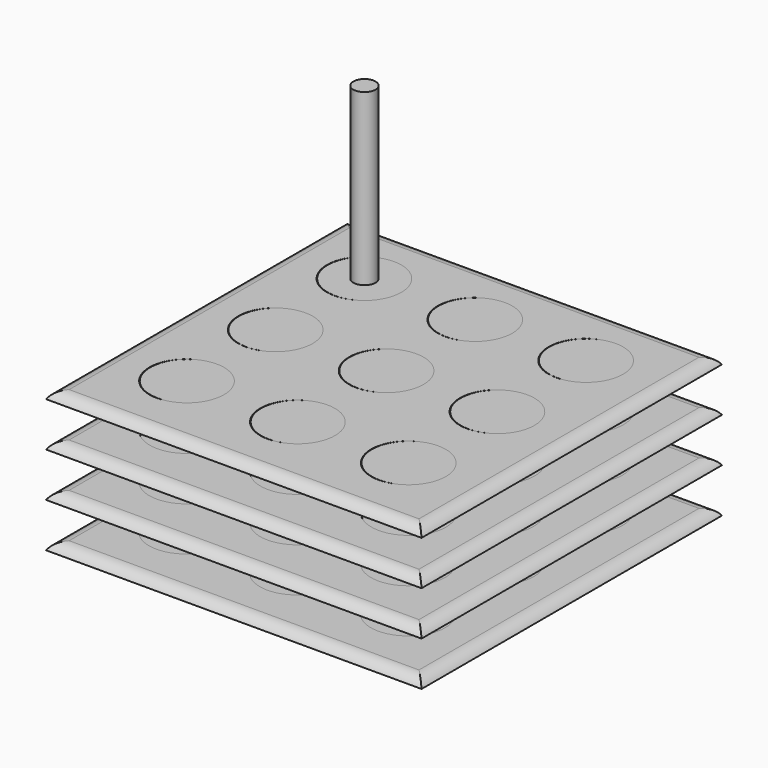
from build123d import *

# Parameters (mm, degrees)
F0_W        = 50.8
F0_H        = 50.8
F1_DEPTH    = 1
F2_T1_DEPTH = 59.4602540378
F2_T3_DEPTH = 59.4602540378
F4_D        = 10
F4_DEPTH    = 1
F4_TIP      = 3.0043030951
F6_R        = 5.0378850753
F7_DEPTH    = 1
F10_R       = 5.0007120409
F11_DEPTH   = 1
F14_R       = 5.0415091702
F15_DEPTH   = 1
F18_R       = 5.001829943
F19_DEPTH   = 1
F20_R       = 1.5
F21_DEPTH   = 40


# Not quite as in the source:
# - a fillet or chamfer that OpenCascade refuses, or shapes differently, is made with other operations: its cross-section is extruded or revolved along the edge and cut away or added


with BuildPart() as f1:
    # F0 (on Top) → F1 (new body)
    with BuildSketch(Plane.XY):
        with Locations((4.2530756999, 25.4)):
            Rectangle(F0_W, F0_H)
    extrude(amount=F1_DEPTH)

    # F2: fillet of radius 2 on 4 edges, made by hand

    # F2_s2 → F2_t1 (cut)
    with BuildSketch(Plane.YZ.offset(-25.477051319)):
        with BuildLine():
            ThreePointArc((0, 0), (0.7320508076, 0.7320508076), (1.7320508076, 1))
            Line((1.7320508076, 1), (0, 1))
            Line((0, 1), (0, 0))
        make_face()
        with BuildLine():
            ThreePointArc((50.8, 0), (50.0679491924, 0.7320508076), (49.0679491924, 1))
            Line((49.0679491924, 1), (50.8, 1))
            Line((50.8, 1), (50.8, 0))
        make_face()
    extrude(amount=F2_T1_DEPTH, mode=Mode.SUBTRACT)

    # F2_s4 → F2_t3 (cut)
    with BuildSketch(Plane.XZ.offset(-55.1301270189)):
        with BuildLine():
            ThreePointArc((29.6530756999, 0), (28.9210248923, 0.7320508076), (27.9210248923, 1))
            Line((27.9210248923, 1), (29.6530756999, 1))
            Line((29.6530756999, 1), (29.6530756999, 0))
        make_face()
        with BuildLine():
            ThreePointArc((-21.1469243001, 0), (-20.4148734925, 0.7320508076), (-19.4148734925, 1))
            Line((-19.4148734925, 1), (-21.1469243001, 1))
            Line((-21.1469243001, 1), (-21.1469243001, 0))
        make_face()
    extrude(amount=F2_T3_DEPTH, mode=Mode.SUBTRACT)

    # F4
    with Locations(Plane.XY.offset(1)):
        with Locations((19.036982879, 41.0148405656), (19.036982879, 26.0148405656), (19.036982879, 11.0148405656), (4.036982879, 11.0148405656), (4.036982879, 26.0148405656), (4.036982879, 41.0148405656), (-10.963017121, 41.0148405656), (-10.963017121, 26.0148405656), (-10.963017121, 11.0148405656)):
            Hole(F4_D / 2, depth=F4_DEPTH)
            with Locations((0, 0, -(F4_DEPTH + F4_TIP / 2))):  # 118° drill point
                Cone(0, F4_D / 2, F4_TIP, mode=Mode.SUBTRACT)


with BuildPart() as f7:
    # F6 (on offset) → F7 (new body)
    with BuildSketch(Plane.XY.offset(1)):
        with Locations((-10.9860114753, 41.0153977573)):
            Circle(F6_R)
    extrude(amount=-F7_DEPTH)


with BuildPart() as f7b:
    # F6 (on offset) → F7, piece 2 (new body)
    with BuildSketch(Plane.XY.offset(1)):
        with Locations((4.0139885247, 41.0153977573)):
            Circle(F6_R)
    extrude(amount=-F7_DEPTH)


with BuildPart() as f7c:
    # F6 (on offset) → F7, piece 3 (new body)
    with BuildSketch(Plane.XY.offset(1)):
        with Locations((19.0139885247, 41.0153977573)):
            Circle(F6_R)
    extrude(amount=-F7_DEPTH)


with BuildPart() as f7d:
    # F6 (on offset) → F7, piece 4 (new body)
    with BuildSketch(Plane.XY.offset(1)):
        with Locations((-10.9860114753, 26.0153977573)):
            Circle(F6_R)
    extrude(amount=-F7_DEPTH)


with BuildPart() as f7e:
    # F6 (on offset) → F7, piece 5 (new body)
    with BuildSketch(Plane.XY.offset(1)):
        with Locations((4.0139885247, 26.0153977573)):
            Circle(F6_R)
    extrude(amount=-F7_DEPTH)


with BuildPart() as f7f:
    # F6 (on offset) → F7, piece 6 (new body)
    with BuildSketch(Plane.XY.offset(1)):
        with Locations((19.0139885247, 26.0153977573)):
            Circle(F6_R)
    extrude(amount=-F7_DEPTH)


with BuildPart() as f7g:
    # F6 (on offset) → F7, piece 7 (new body)
    with BuildSketch(Plane.XY.offset(1)):
        with Locations((-10.9860114753, 11.0153977573)):
            Circle(F6_R)
    extrude(amount=-F7_DEPTH)


with BuildPart() as f7h:
    # F6 (on offset) → F7, piece 8 (new body)
    with BuildSketch(Plane.XY.offset(1)):
        with Locations((4.0139885247, 11.0153977573)):
            Circle(F6_R)
    extrude(amount=-F7_DEPTH)


with BuildPart() as f7i:
    # F6 (on offset) → F7, piece 9 (new body)
    with BuildSketch(Plane.XY.offset(1)):
        with Locations((19.0139885247, 11.0153977573)):
            Circle(F6_R)
    extrude(amount=-F7_DEPTH)


with BuildPart() as f8_1:
    # F8: copy of F1
    add(f1.part.moved(Location((0, 0, 6))))


with BuildPart() as f11:
    # F10 (on offset) → F11 (new body)
    with BuildSketch(Plane.XY.offset(7)):
        with Locations((19.0628959137, 40.9449415705)):
            Circle(F10_R)
    extrude(amount=-F11_DEPTH)


with BuildPart() as f11b:
    # F10 (on offset) → F11, piece 2 (new body)
    with BuildSketch(Plane.XY.offset(7)):
        with Locations((19.0628959137, 25.9449415705)):
            Circle(F10_R)
    extrude(amount=-F11_DEPTH)


with BuildPart() as f11c:
    # F10 (on offset) → F11, piece 3 (new body)
    with BuildSketch(Plane.XY.offset(7)):
        with Locations((19.0628959137, 10.9449415705)):
            Circle(F10_R)
    extrude(amount=-F11_DEPTH)


with BuildPart() as f11d:
    # F10 (on offset) → F11, piece 4 (new body)
    with BuildSketch(Plane.XY.offset(7)):
        with Locations((4.0628959137, 40.9449415705)):
            Circle(F10_R)
    extrude(amount=-F11_DEPTH)


with BuildPart() as f11e:
    # F10 (on offset) → F11, piece 5 (new body)
    with BuildSketch(Plane.XY.offset(7)):
        with Locations((4.0628959137, 25.9449415705)):
            Circle(F10_R)
    extrude(amount=-F11_DEPTH)


with BuildPart() as f11f:
    # F10 (on offset) → F11, piece 6 (new body)
    with BuildSketch(Plane.XY.offset(7)):
        with Locations((4.0628959137, 10.9449415705)):
            Circle(F10_R)
    extrude(amount=-F11_DEPTH)


with BuildPart() as f11g:
    # F10 (on offset) → F11, piece 7 (new body)
    with BuildSketch(Plane.XY.offset(7)):
        with Locations((-10.9371040863, 10.9449415705)):
            Circle(F10_R)
    extrude(amount=-F11_DEPTH)


with BuildPart() as f11h:
    # F10 (on offset) → F11, piece 8 (new body)
    with BuildSketch(Plane.XY.offset(7)):
        with Locations((-10.9371040863, 25.9449415705)):
            Circle(F10_R)
    extrude(amount=-F11_DEPTH)


with BuildPart() as f11i:
    # F10 (on offset) → F11, piece 9 (new body)
    with BuildSketch(Plane.XY.offset(7)):
        with Locations((-10.9371040863, 40.9449415705)):
            Circle(F10_R)
    extrude(amount=-F11_DEPTH)


with BuildPart() as f12_1:
    # F12: copy of F8_1
    add(f8_1.part.moved(Location((0, 0, 6))))


with BuildPart() as f15:
    # F14 (on offset) → F15 (new body)
    with BuildSketch(Plane.XY.offset(13)):
        with Locations((-10.9040877064, 41.0306417219)):
            Circle(F14_R)
    extrude(amount=-F15_DEPTH)


with BuildPart() as f15b:
    # F14 (on offset) → F15, piece 2 (new body)
    with BuildSketch(Plane.XY.offset(13)):
        with Locations((-10.9040877064, 26.0306417219)):
            Circle(F14_R)
    extrude(amount=-F15_DEPTH)


with BuildPart() as f15c:
    # F14 (on offset) → F15, piece 3 (new body)
    with BuildSketch(Plane.XY.offset(13)):
        with Locations((-10.9040877064, 11.0306417219)):
            Circle(F14_R)
    extrude(amount=-F15_DEPTH)


with BuildPart() as f15d:
    # F14 (on offset) → F15, piece 4 (new body)
    with BuildSketch(Plane.XY.offset(13)):
        with Locations((4.0959122936, 41.0306417219)):
            Circle(F14_R)
    extrude(amount=-F15_DEPTH)


with BuildPart() as f15e:
    # F14 (on offset) → F15, piece 5 (new body)
    with BuildSketch(Plane.XY.offset(13)):
        with Locations((4.0959122936, 26.0306417219)):
            Circle(F14_R)
    extrude(amount=-F15_DEPTH)


with BuildPart() as f15f:
    # F14 (on offset) → F15, piece 6 (new body)
    with BuildSketch(Plane.XY.offset(13)):
        with Locations((4.0959122936, 11.0306417219)):
            Circle(F14_R)
    extrude(amount=-F15_DEPTH)


with BuildPart() as f15g:
    # F14 (on offset) → F15, piece 7 (new body)
    with BuildSketch(Plane.XY.offset(13)):
        with Locations((19.0959122936, 41.0306417219)):
            Circle(F14_R)
    extrude(amount=-F15_DEPTH)


with BuildPart() as f15h:
    # F14 (on offset) → F15, piece 8 (new body)
    with BuildSketch(Plane.XY.offset(13)):
        with Locations((19.0959122936, 26.0306417219)):
            Circle(F14_R)
    extrude(amount=-F15_DEPTH)


with BuildPart() as f15i:
    # F14 (on offset) → F15, piece 9 (new body)
    with BuildSketch(Plane.XY.offset(13)):
        with Locations((19.0959122936, 11.0306417219)):
            Circle(F14_R)
    extrude(amount=-F15_DEPTH)


with BuildPart() as f16_1:
    # F16: copy of F12_1
    add(f12_1.part.moved(Location((0, 0, 6))))


with BuildPart() as f19:
    # F18 (on offset) → F19 (new body)
    with BuildSketch(Plane.XY.offset(19)):
        with Locations((-10.9060970124, 41.0428672295)):
            Circle(F18_R)
    extrude(amount=-F19_DEPTH)


with BuildPart() as f19b:
    # F18 (on offset) → F19, piece 2 (new body)
    with BuildSketch(Plane.XY.offset(19)):
        with Locations((-10.9060970124, 26.0428672295)):
            Circle(F18_R)
    extrude(amount=-F19_DEPTH)


with BuildPart() as f19c:
    # F18 (on offset) → F19, piece 3 (new body)
    with BuildSketch(Plane.XY.offset(19)):
        with Locations((-10.9060970124, 11.0428672295)):
            Circle(F18_R)
    extrude(amount=-F19_DEPTH)


with BuildPart() as f19d:
    # F18 (on offset) → F19, piece 4 (new body)
    with BuildSketch(Plane.XY.offset(19)):
        with Locations((4.0939029876, 41.0428672295)):
            Circle(F18_R)
    extrude(amount=-F19_DEPTH)


with BuildPart() as f19e:
    # F18 (on offset) → F19, piece 5 (new body)
    with BuildSketch(Plane.XY.offset(19)):
        with Locations((4.0939029876, 26.0428672295)):
            Circle(F18_R)
    extrude(amount=-F19_DEPTH)


with BuildPart() as f19f:
    # F18 (on offset) → F19, piece 6 (new body)
    with BuildSketch(Plane.XY.offset(19)):
        with Locations((4.0939029876, 11.0428672295)):
            Circle(F18_R)
    extrude(amount=-F19_DEPTH)


with BuildPart() as f19g:
    # F18 (on offset) → F19, piece 7 (new body)
    with BuildSketch(Plane.XY.offset(19)):
        with Locations((19.0939029876, 41.0428672295)):
            Circle(F18_R)
    extrude(amount=-F19_DEPTH)


with BuildPart() as f19h:
    # F18 (on offset) → F19, piece 8 (new body)
    with BuildSketch(Plane.XY.offset(19)):
        with Locations((19.0939029876, 26.0428672295)):
            Circle(F18_R)
    extrude(amount=-F19_DEPTH)


with BuildPart() as f19i:
    # F18 (on offset) → F19, piece 9 (new body)
    with BuildSketch(Plane.XY.offset(19)):
        with Locations((19.0939029876, 11.0428672295)):
            Circle(F18_R)
    extrude(amount=-F19_DEPTH)


with BuildPart() as f21:
    # F20 (on offset) → F21 (new body)
    with BuildSketch(Plane.XY.offset(19)):
        with Locations((-10.9060970124, 41.0428672295)):
            Circle(F20_R)
    extrude(amount=F21_DEPTH)


with BuildPart() as f21_1:
    # F22: moved
    add(f21.part.moved(Location((0, 0, -17))))


solid = Compound([f1.part, f7.part, f7b.part, f7c.part, f7d.part, f7e.part, f7f.part, f7g.part, f7h.part, f7i.part, f8_1.part, f11.part, f11b.part, f11c.part, f11d.part, f11e.part, f11f.part, f11g.part, f11h.part, f11i.part, f12_1.part, f15.part, f15b.part, f15c.part, f15d.part, f15e.part, f15f.part, f15g.part, f15h.part, f15i.part, f16_1.part, f19.part, f19b.part, f19c.part, f19d.part, f19e.part, f19f.part, f19g.part, f19h.part, f19i.part, f21_1.part])
